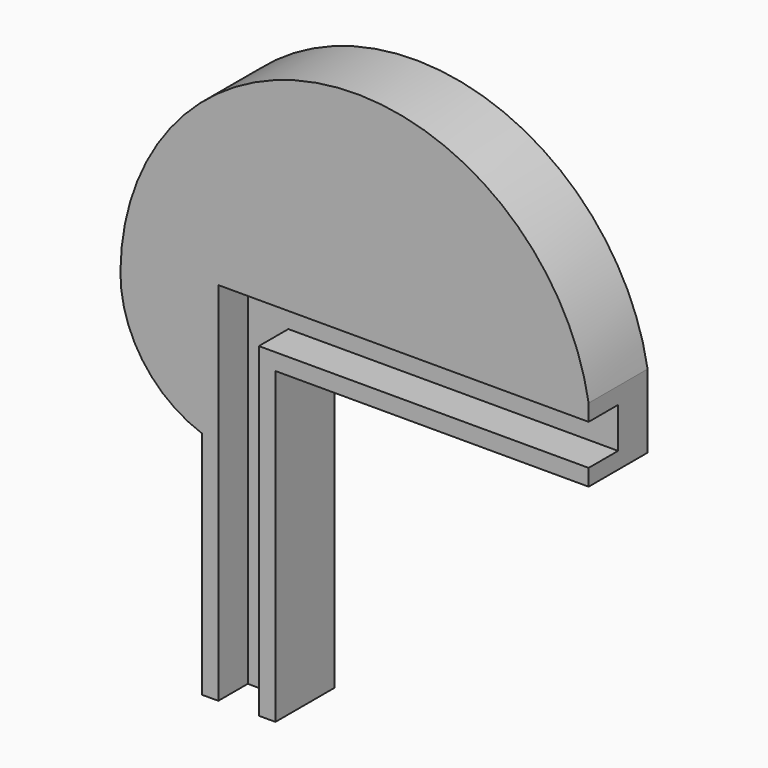
from build123d import *

# Parameters (mm, degrees)
F1_DEPTH = 10
F3_DEPTH = 5


# Not quite as in the source:
# - a feature names something its author has since deleted; it is built from what else it names


with BuildPart() as f1:
    # F0 (on Front) → F1 (new body)
    with BuildSketch(Plane.XZ):
        with BuildLine():
            Line((4.5435639801, -4.8811539246), (47.0578219503, -4.8811539246))
            Line((47.0578219503, -4.8811539246), (47.0578219503, 5.1188460754))
            ThreePointArc((47.0578219503, 5.1188460754), (13.0237482483, 31.7276460361), (-16.4989304836, 0.1878640363))
            ThreePointArc((-16.4989304836, 0.1878640363), (-13.5129700245, -9.4683494399), (-5.4564360199, -15.5716828237))
            Line((-5.4564360199, -15.5716828237), (-5.4564360199, -46.8141730692))
            Line((-5.4564360199, -46.8141730692), (4.5435639801, -46.8141730692))
            Line((4.5435639801, -46.8141730692), (4.5435639801, -4.8811539246))
        make_face()
    extrude(amount=F1_DEPTH)

    # F2 (on face) → F3 (cut)
    with BuildSketch(Plane.XZ.offset(10)):
        Polygon((47.0578219503, -2.6311539246), (47.0578219503, 2.8688460754), (-3.2064360199, 2.8688460754), (-3.2064360199, -2.6311539246), (-3.2064360199, -46.8141730692), (2.2935639801, -46.8141730692), (2.2935639801, -2.6311539246), align=None)
    extrude(amount=-F3_DEPTH, mode=Mode.SUBTRACT)


solid = f1.part
